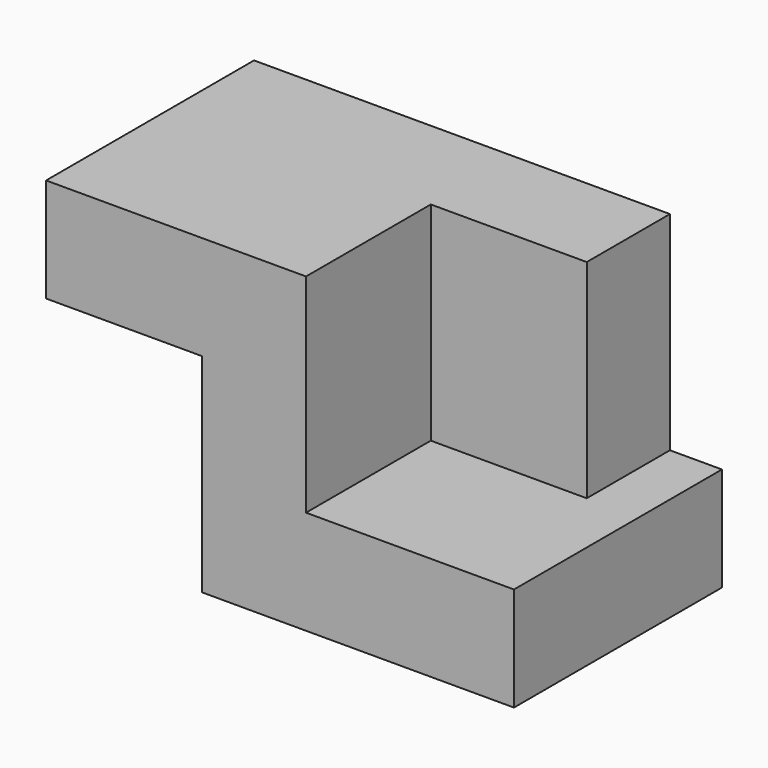
from build123d import *

# Parameters (mm, degrees)
F1_DEPTH = 63.5
F2_W     = 38.1
F2_H     = 25.4
F3_DEPTH = 50.8


# Not quite as in the source:
# - a feature names something its author has since deleted; it is built from what else it names


with BuildPart() as f1:
    # F0 (on Front) → F1 (new body)
    with BuildSketch(Plane.XZ):
        Polygon((-30.3928350806, -50.8), (45.8071649194, -50.8), (45.8071649194, -25.4), (-4.9928350806, -25.4), (-4.9928350806, 25.4), (-68.4928350806, 25.4), (-68.4928350806, 0), (-30.3928350806, 0), align=None)
    extrude(amount=F1_DEPTH)

    # F2 (on face) → F3 (join)
    with BuildSketch(Plane.XY.offset(-25.4)):
        with Locations((14.0571649194, -12.7)):
            Rectangle(F2_W, F2_H)
    extrude(amount=F3_DEPTH)


solid = f1.part
